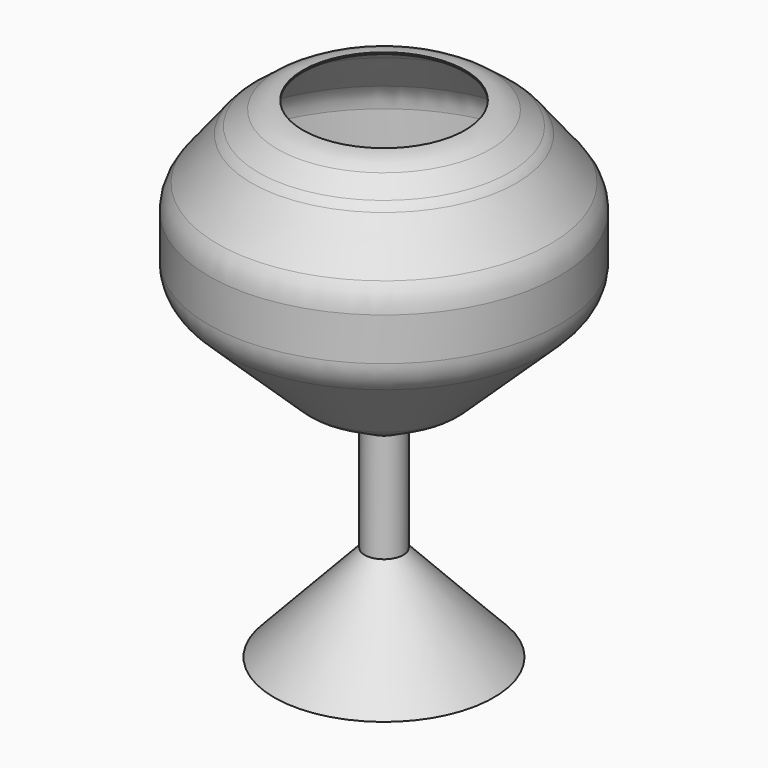
from build123d import *

# Parameters (mm, degrees)
F2_T = 0.254


# Not quite as in the source:
# - a shell that OpenCascade refuses in one call is made with other operations: the cavity is built on its own and cut out
# - a feature names something its author has since deleted; it is built from what else it names


with BuildPart() as f1:
    # F0 (on Front) → F1 (revolve)
    with BuildSketch(Plane.XZ):
        with BuildLine():
            Line((-3.0112911481, 31.8550616503), (-3.0112911481, 14.9488672614))
            Line((-3.0112911481, 14.9488672614), (-17.0688, 0))
            Line((-17.0688, 0), (0, 0))
            Line((0, 0), (0, 76.0556012392))
            Line((0, 76.0556012392), (-12.6169178095, 76.228944836))
            ThreePointArc((-12.6169178095, 76.228944836), (-14.7075461422, 75.9052317699), (-16.5758116747, 74.9127092893))
            Line((-16.5758116747, 74.9127092893), (-19.5062669903, 72.6585163811))
            ThreePointArc((-19.5062669903, 72.6585163811), (-20.0880647436, 72.1518528829), (-20.6041254437, 71.57837413))
            Line((-20.6041254437, 71.57837413), (-25.8698135255, 64.9586474103))
            ThreePointArc((-25.8698135255, 64.9586474103), (-26.8952491924, 63.0991932265), (-27.2502955049, 61.005624435))
            Line((-27.2502955049, 61.005624435), (-27.2502955049, 54.34028509))
            ThreePointArc((-27.2502955049, 54.34028509), (-26.7348850464, 51.8342793274), (-25.2723223137, 49.735083511))
            Line((-25.2723223137, 49.735083511), (-11.7529370155, 36.9002240705))
            ThreePointArc((-11.7529370155, 36.9002240705), (-11.1278091674, 36.3787066033), (-10.4410949941, 35.9414550289))
            Line((-10.4410949941, 35.9414550289), (-3.0112911481, 31.8550616503))
        make_face()
    revolve(axis=Axis((0, 0, 38.0278006196), (0, 0, -1)))

    # F2: shell of thickness 0.254, made by hand


with BuildPart() as f2_core1:
    # F2_t2: copy of F1
    add(f1.part)

    # the walls: a layer under each face that stays
    f2_faces = [f2_core1.faces().sort_by_distance(p)[0] for p in [
        (3.0112911481, 0, 23.4019644558),
        (10.0400455741, 0, 7.4744336307),
        (14.7075461422, 0, 75.9052317699),
        (18.0410393325, 0, 73.7856128352),
        (20.0880647436, 0, 72.1518528829),
        (23.2369694846, 0, 68.2685107702),
        (26.8952491924, 0, 63.0991932265),
        (27.2502955049, 0, 57.6729547625),
        (26.7348850464, 0, 51.8342793274),
        (18.5126296646, 0, 43.3176537907),
        (11.1278091674, 0, 36.3787066033),
        (6.7261930711, 0, 33.8982583396),
    ]]
    thicken(f2_faces, amount=-F2_T, mode=Mode.SUBTRACT)

    # F2_s3 → F2_t4 (revolve, cut)
    with BuildSketch(Plane.XZ):
        Polygon((-3.0150552221, 31.852836062), (-2.7572911481, 31.8550616503), (-2.7572911481, 32.005244518), (-2.8888837566, 32.0776204751), align=None)
    revolve(axis=Axis((0, 0, 31.8550616503), (0, 0, -1)), mode=Mode.SUBTRACT)

    # F2_s5 → F2_t6 (revolve, cut)
    with BuildSketch(Plane.XZ):
        Polygon((-3.0156815181, 14.9506072991), (-2.7572911481, 14.9488672614), (-2.7572911481, 14.8481993064), (-2.8262541531, 14.7748634958), align=None)
    revolve(axis=Axis((0, 0, 14.9488672614), (0, 0, -1)), mode=Mode.SUBTRACT)


with BuildPart() as f1_1:
    add(f1.part)

    # what is left inside the walls is the cavity
    f2_cavity = [f2_core1.part.solids().sort_by_distance(p)[0] for p in [
        (20.589231, 0, 45.642847),
    ]]
    add(f2_cavity, mode=Mode.SUBTRACT)


solid = f1_1.part
